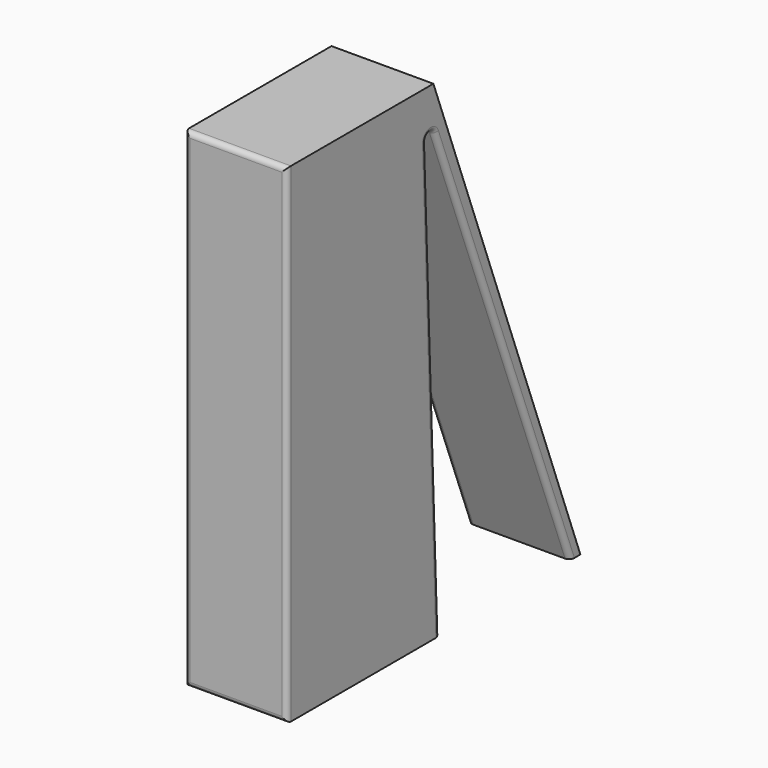
from build123d import *

# Parameters (mm, degrees)
F0_W     = 254
F0_H     = 1219.2
F1_DEPTH = 914.4
F3_DEPTH = 254.001
F5_DEPTH = 254.001
F6_F1_R  = 12.7
F6_F2_R  = 12.7


with BuildPart() as f1:
    # F0 (on Front) → F1 (new body)
    with BuildSketch(Plane.XZ):
        with Locations((-127, 609.6)):
            Rectangle(F0_W, F0_H)
    extrude(amount=F1_DEPTH)

    # F2 (on Right) → F3 (cut, through all)
    with BuildSketch(Plane.YZ):
        Polygon((-462.4002873898, 1231.0378551483), (0, 0), (0, 1231.0378551483), align=None)
    extrude(amount=-F3_DEPTH, mode=Mode.SUBTRACT)

    # F4 (on Right) → F5 (cut, through all)
    with BuildSketch(Plane.YZ):
        Polygon((-437.4758601189, 0), (-32.0333614945, 0), (-481.8673729897, 1177.9962778091), align=None)
    extrude(amount=-F5_DEPTH, mode=Mode.SUBTRACT)

    # F6: fillet of radius 12.7 on 8 edges, made by hand

    # F6_f1
    f6_f1_edges = [f1.edges().sort_by_distance(p)[0] for p in [
        (-127, -481.8673729897, 1177.9962778091),
    ]]
    fillet(f6_f1_edges, radius=F6_F1_R)

    # F6_f2
    f6_f2_edges = [f1.edges().sort_by_distance(p)[0] for p in [
        (-127, -914.4, 0),
        (0, -914.4, 609.6),
        (-127, -914.4, 1219.2),
        (-254, -914.4, 609.6),
        (0, -458.2226343973, 550.5471946336),
        (-127, -437.4758601189, 0),
        (-254, -458.2226343973, 550.5471946336),
        (-254, -468.8167042617, 1114.0163928436),
        (0, -468.8167042617, 1114.0163928436),
    ]]
    fillet(f6_f2_edges, radius=F6_F2_R)


solid = f1.part
